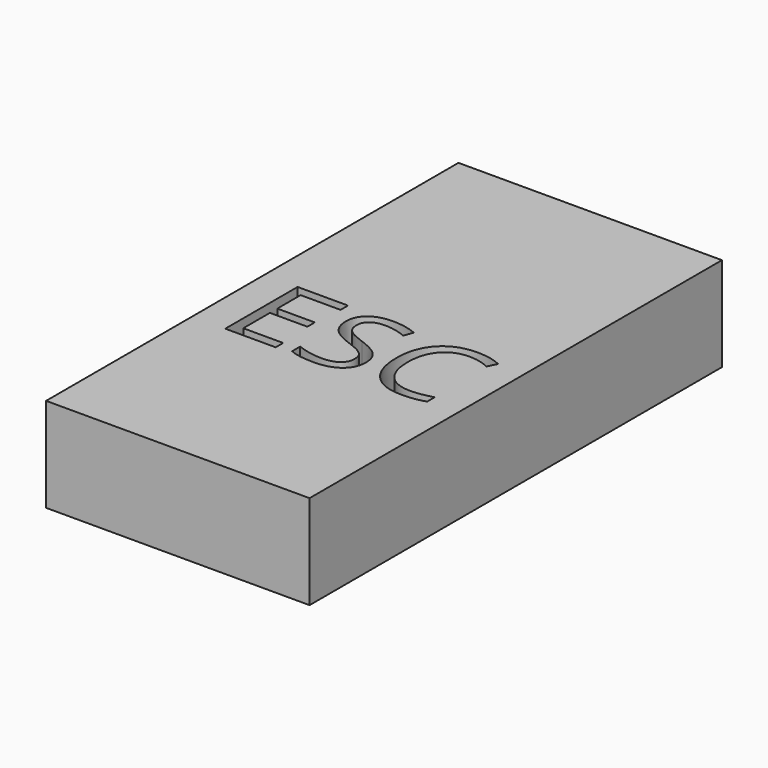
from build123d import *

# Parameters (mm, degrees)
F0_W         = 17.62
F0_H         = 34.47
F1_DEPTH     = 6.3
F2_TEXT_SIZE = 8.4700899947
F3_DEPTH     = 3


# Not quite as in the source:
# - Text() gives the source's letters only with a copy of the font that has no kerning and outlines rounded to 1/6400 em; it was checked with that copy


with BuildPart() as f1:
    # F0 (on Top) → F1 (new body)
    with BuildSketch(Plane.XY):
        Rectangle(F0_W, F0_H)
    extrude(amount=F1_DEPTH)

    # F2 (on face) → F3 (cut)
    with BuildSketch(Plane.XY.offset(6.3)):
        with Locations((-7.4322353344, -5.0185759566)):
            Text('ESC', F2_TEXT_SIZE, font='Open Sans', text_align=(TextAlign.LEFT, TextAlign.BOTTOM))
    extrude(amount=-F3_DEPTH, mode=Mode.SUBTRACT)


solid = f1.part
